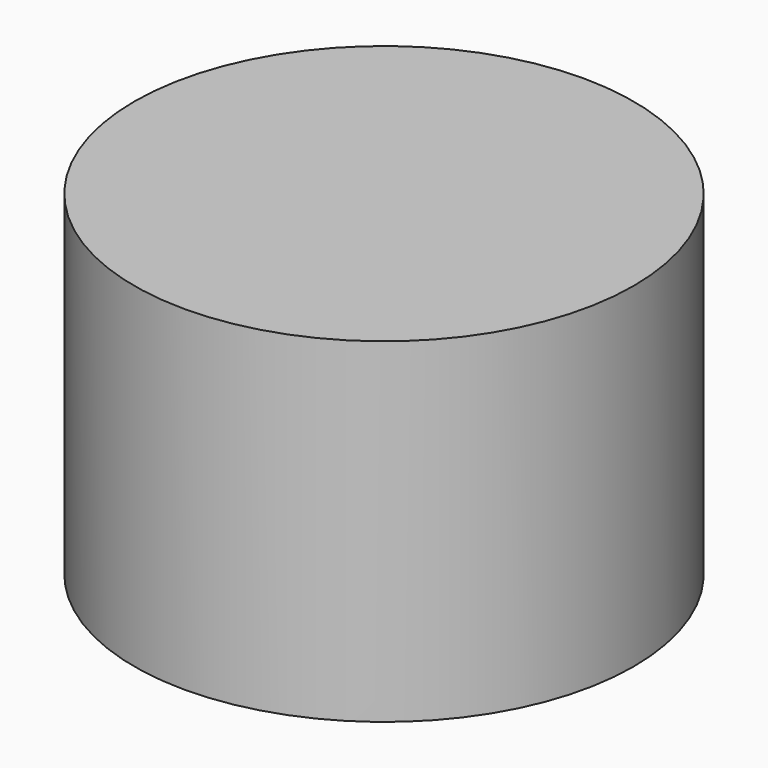
from build123d import *

# Parameters (mm, degrees)
F3_R     = 14.9
F5_DEPTH = 20


# Not quite as in the source:
# - the program builds the solid bodies; features that only make, move or delete a surface that nothing else refers to are left out


with BuildPart() as f5:
    # F3 (on Top) → F5 (new body)
    with BuildSketch(Plane.XY):
        with Locations((-30.0935078294, -6.574e-06)):
            Circle(F3_R)
    extrude(amount=F5_DEPTH)


solid = f5.part
